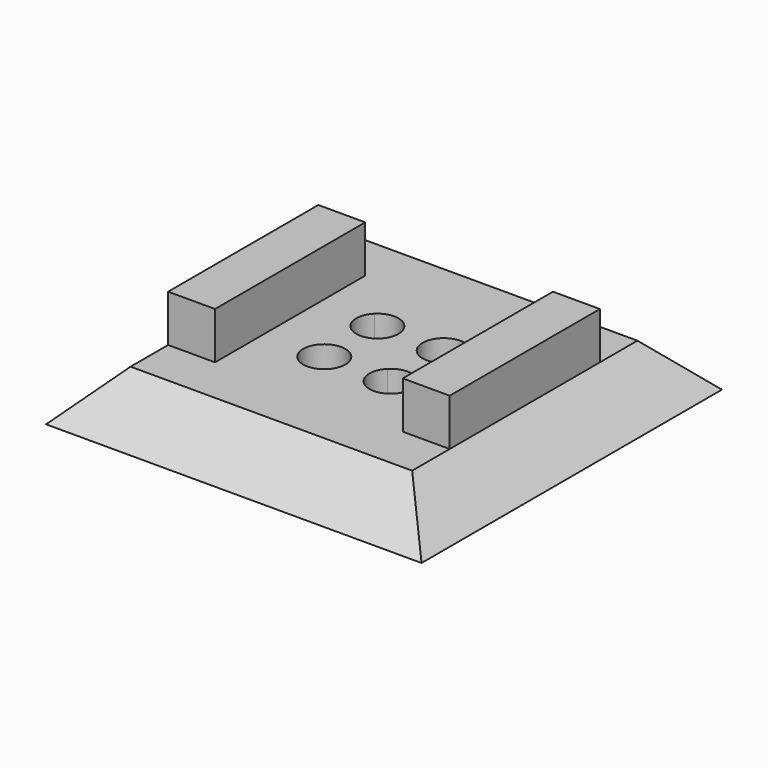
from build123d import *

# Parameters (mm, degrees)
F0_W     = 80
F0_H     = 80
F1_DEPTH = 10
F2_SIZE2 = 9.99999
F2_SIZE  = 9.99999
F3_W     = 10
F3_H     = 40
F4_DEPTH = 10
F6_DEPTH = 8


# Not quite as in the source:
# - a fillet or chamfer is up to 0.001 mm smaller than in the source, because OpenCascade refuses the exact size


with BuildPart() as f1:
    # F0 (on Top) → F1 (new body)
    with BuildSketch(Plane.XY):
        Rectangle(F0_W, F0_H)
    extrude(amount=F1_DEPTH)

    # F2 (size 10 and 10 in the source; OpenCascade refuses exactly that, so slightly less here)
    f2_edges = [f1.edges().sort_by_distance(p)[0] for p in [
        (0, 40, 10),
        (-40, 0, 10),
        (0, -40, 10),
        (40, 0, 10),
    ]]
    chamfer(f2_edges, length=F2_SIZE, length2=F2_SIZE2)

    # F3 (on face) → F4 (join)
    with BuildSketch(Plane.XY.offset(10)):
        with Locations((25, 0)):
            Rectangle(F3_W, F3_H)
        with Locations((-25, 0)):
            Rectangle(F3_W, F3_H)
    extrude(amount=F4_DEPTH)

    # F5 (on face) → F6 (cut)
    with BuildSketch(Plane.XY.offset(10)):
        with BuildLine():
            Line((-3.8890872965, -3.8890872965), (-10.2530483272, -10.2530483272))
            ThreePointArc((-10.2530483272, -10.2530483272), (-5.3489923662, -11.2285257082), (-2.5710678119, -7.0710678119))
            ThreePointArc((-2.5710678119, -7.0710678119), (-2.9136099156, -5.3489923662), (-3.8890872965, -3.8890872965))
        make_face()
        with BuildLine():
            Line((3.8890872965, 3.8890872965), (10.2530483272, 10.2530483272))
            ThreePointArc((10.2530483272, 10.2530483272), (3.8890872965, 10.2530483272), (3.8890872965, 3.8890872965))
        make_face()
        with BuildLine():
            ThreePointArc((-2.5710678119, 7.0710678119), (-5.3489923662, 11.2285257082), (-10.2530483272, 10.2530483272))
            Line((-10.2530483272, 10.2530483272), (-3.8890872965, 3.8890872965))
            ThreePointArc((-3.8890872965, 3.8890872965), (-2.9136099156, 5.3489923662), (-2.5710678119, 7.0710678119))
        make_face()
        with BuildLine():
            ThreePointArc((11.5710678119, 7.0710678119), (11.2285257082, 8.7931432575), (10.2530483272, 10.2530483272))
            Line((10.2530483272, 10.2530483272), (3.8890872965, 3.8890872965))
            ThreePointArc((3.8890872965, 3.8890872965), (8.7931432575, 2.9136099156), (11.5710678119, 7.0710678119))
        make_face()
        with BuildLine():
            ThreePointArc((3.8890872965, -3.8890872965), (3.8890872965, -10.2530483272), (10.2530483272, -10.2530483272))
            Line((10.2530483272, -10.2530483272), (3.8890872965, -3.8890872965))
        make_face()
        with BuildLine():
            Line((-3.8890872965, 3.8890872965), (-10.2530483272, 10.2530483272))
            ThreePointArc((-10.2530483272, 10.2530483272), (-10.2530483272, 3.8890872965), (-3.8890872965, 3.8890872965))
        make_face()
        with BuildLine():
            ThreePointArc((-3.8890872965, -3.8890872965), (-10.2530483272, -3.8890872965), (-10.2530483272, -10.2530483272))
            Line((-10.2530483272, -10.2530483272), (-3.8890872965, -3.8890872965))
        make_face()
        with BuildLine():
            Line((3.8890872965, -3.8890872965), (10.2530483272, -10.2530483272))
            ThreePointArc((10.2530483272, -10.2530483272), (11.2285257082, -8.7931432575), (11.5710678119, -7.0710678119))
            ThreePointArc((11.5710678119, -7.0710678119), (8.7931432575, -2.9136099156), (3.8890872965, -3.8890872965))
        make_face()
    extrude(amount=-F6_DEPTH, mode=Mode.SUBTRACT)


solid = f1.part
